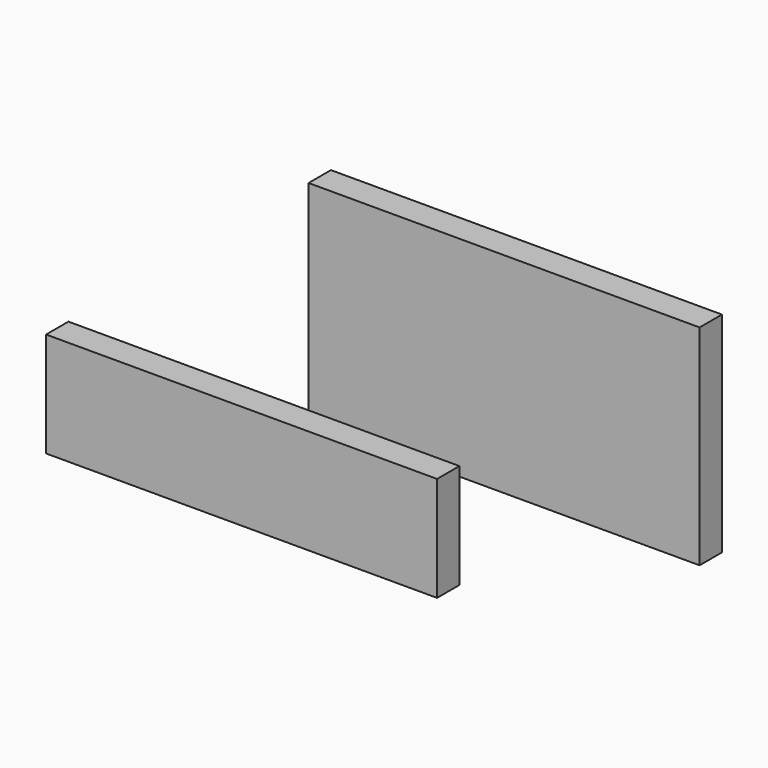
from build123d import *

# Parameters (mm, degrees)
F0_W     = 5600
F0_H     = 400
F1_DEPTH = 1500
F2_DEPTH = 3000


# Not quite as in the source:
# - the program builds the solid bodies; features that only make, move or delete a surface that nothing else refers to are left out


with BuildPart() as f1:
    # F0 (on Top) → F1 (new body)
    with BuildSketch(Plane.XY):
        with Locations((-4300, -2350)):
            Rectangle(F0_W, F0_H)
    extrude(amount=-F1_DEPTH)


with BuildPart() as f2:
    # F0 (on Top) → F2 (new body)
    with BuildSketch(Plane.XY):
        with Locations((-4300, 2350)):
            Rectangle(F0_W, F0_H)
    extrude(amount=-F2_DEPTH)


solid = Compound([f1.part, f2.part])
